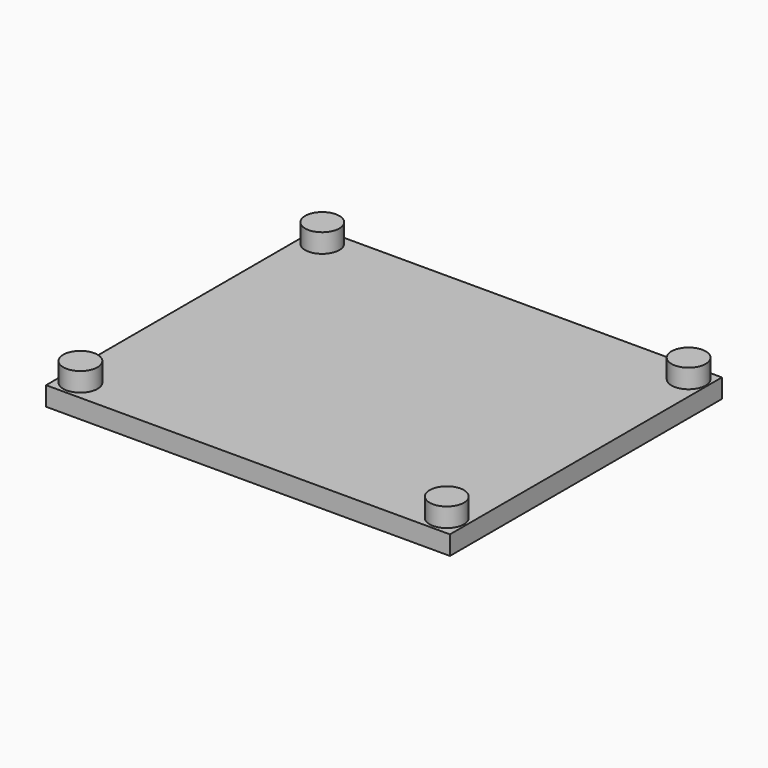
from build123d import *

# Parameters (mm, degrees)
F0_R     = 2.25
F1_DEPTH = 5
F0_W     = 53.1
F0_H     = 44.7
F2_DEPTH = 2.5


# Not quite as in the source:
# - the program builds the solid bodies; features that only make, move or delete a surface that nothing else refers to are left out


with BuildPart() as f1:
    # F0 (on Top) → F1 (new body)
    with BuildSketch(Plane.XY):
        with Locations((24.1313669831, 19.8986493051)):
            Circle(F0_R)
    extrude(amount=F1_DEPTH)


with BuildPart() as f1b:
    # F0 (on Top) → F1, piece 2 (new body)
    with BuildSketch(Plane.XY):
        with Locations((-24.0537095815, 19.9159570038)):
            Circle(F0_R)
    extrude(amount=F1_DEPTH)


with BuildPart() as f1c:
    # F0 (on Top) → F1, piece 3 (new body)
    with BuildSketch(Plane.XY):
        with Locations((-24.1623297334, -19.694061164)):
            Circle(F0_R)
    extrude(amount=F1_DEPTH)


with BuildPart() as f1d:
    # F0 (on Top) → F1, piece 4 (new body)
    with BuildSketch(Plane.XY):
        with Locations((24.0227468312, -19.7113688628)):
            Circle(F0_R)
    extrude(amount=F1_DEPTH)


with BuildPart() as f2:
    # F0 (on Top) → F2 (new body)
    with BuildSketch(Plane.XY):
        Rectangle(F0_W, F0_H)
        with Locations((-24.1623297334, -19.694061164)):
            Circle(F0_R, mode=Mode.SUBTRACT)
        with Locations((24.0227468312, -19.7113688628)):
            Circle(F0_R, mode=Mode.SUBTRACT)
        with Locations((-24.0537095815, 19.9159570038)):
            Circle(F0_R, mode=Mode.SUBTRACT)
        with Locations((24.1313669831, 19.8986493051)):
            Circle(F0_R, mode=Mode.SUBTRACT)
    extrude(amount=F2_DEPTH)


solid = Compound([f1.part, f1b.part, f1c.part, f1d.part, f2.part])
